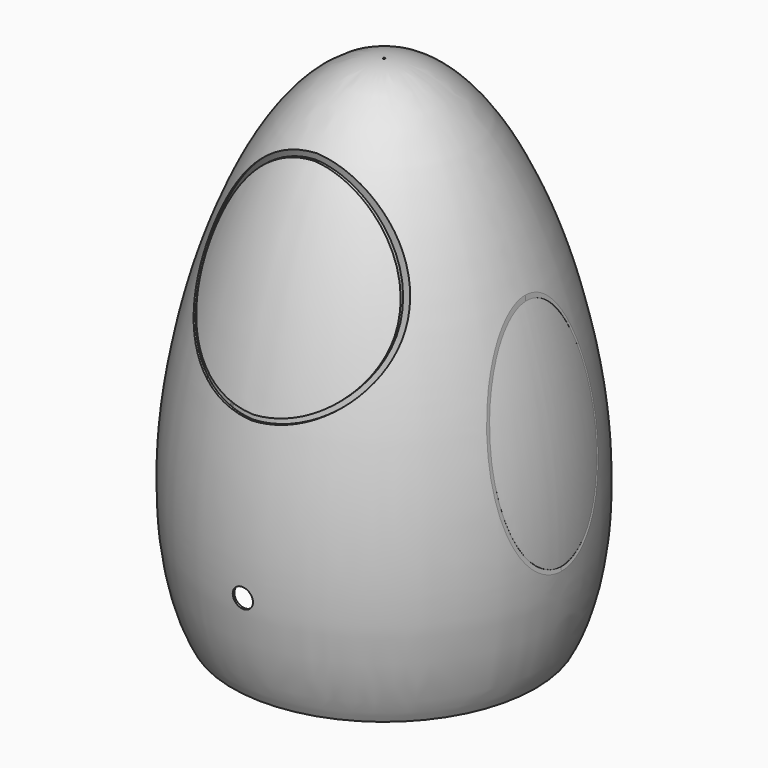
from build123d import *

# Parameters (mm, degrees)
F6_DEPTH       = 176.0365687371
F7_R           = 20
F8_DEPTH       = 15
F10_DEPTH      = 176.0365687371
F10_DEPTH_BACK = 176.0365687371
F12_DEPTH      = 176.0365687371
F12_DEPTH_BACK = 176.0365687371
F13_R          = 10
F14_DEPTH      = 100


# Not quite as in the source:
# - the dataset's text gives a spline's control points without its knots; the knots are read off the source's solid
# - the program builds the solid bodies; features that only make, move or delete a surface that nothing else refers to are left out


with BuildPart() as f4:
    # F2 (on Front) → F4 (revolve)
    with BuildSketch(Plane.XZ):
        with BuildLine():
            add(Edge.make_bspline(
                [(1, 449.0443005306), (80.1100924551, 451.0782588519), (193.5026632526, 197.5216639229), (177.718595848, 0), (150, -50.9556994694)],
                knots=[0, 0, 0, 0, 0.5180034602, 1, 1, 1, 1], degree=3))
            Line((1, 449.0443005306), (1.0514039698, 447.0449612318))
            add(Edge.make_bspline(
                [(1.0514039698, 447.0449612318), (5.6889924562, 447.1641958503), (14.8146657678, 446.4599738755), (28.0818566532, 442.7588814458), (40.9340638175, 436.5780096507), (57.4933039947, 425.253477856), (77.0343246982, 405.7570843458), (98.3770754656, 375.3396271098), (117.4020772089, 339.4781493047), (131.1745767843, 306.3735527905), (140.8608088078, 278.7467501585), (147.4397218669, 257.6520230515), (153.3131918368, 236.3794941135), (157.6036419872, 218.6684679305), (160.6640307325, 204.6072717881), (163.4728613383, 190.6522845028), (166.5161124872, 173.4285279629), (169.4361062201, 153.1618789749), (172.3750814452, 126.7445649885), (174.3001264236, 94.9854795873), (173.9432956348, 59.3073823577), (171.0522793788, 26.4763680651), (165.7627686174, -3.090947369), (158.216194357, -28.9750937643), (151.7820830163, -43.4942412252), (148.2431168154, -50)],
                knots=[0, 0, 0, 0, 0.03125, 0.0625, 0.09375, 0.125, 0.1875, 0.25, 0.3125, 0.375, 0.40625, 0.4375, 0.46875, 0.5, 0.515625, 0.53125, 0.5625, 0.59375, 0.625, 0.6875, 0.75, 0.8125, 0.875, 0.9375, 1, 1, 1, 1], degree=3))
            Line((148.2431168154, -50), (150, -50.9556994694))
        make_face()
    revolve(axis=Axis((0, 0, 140.6808644533), (0, 0, 1)))

    # F5 (on Front) → F6 (cut, through all)
    with BuildSketch(Plane.XZ):
        with BuildLine():
            add(Edge.make_bspline(
                [(0, 400), (59.0140521526, 398.2927203178), (143.2820959516, 269.3665802261), (55.2223846316, 202.2753804922), (0, 200)],
                knots=[0, 0, 0, 0, 0.5248109679, 1, 1, 1, 1], degree=3))
            add(Edge.make_bspline(
                [(0, 400), (-59.0140521526, 398.2927203178), (-143.2820959516, 269.3665802261), (-55.2223846316, 202.2753804922), (0, 200)],
                knots=[0, 0, 0, 0, 0.5248109679, 1, 1, 1, 1], degree=3))
        make_face()
        with BuildLine():
            add(Edge.make_bspline(
                [(-0.0001205983, 394.9977653066), (-6.5310531824, 394.7960276482), (-19.2521705838, 392.663716092), (-37.0198522817, 384.9642174164), (-53.1715953389, 373.423361096), (-67.2769986996, 358.8303413408), (-78.945849914, 342.0125314277), (-86.3298122589, 326.8622632752), (-90.6611195591, 314.5041209951), (-93.0823387791, 305.229555905), (-94.6395134009, 296.0625109198), (-95.189746261, 288.6086395993), (-95.1680818457, 282.8120957412), (-94.8339775011, 277.1489767391), (-93.8311621578, 270.3054768515), (-91.7383515242, 262.4779212136), (-87.8135974939, 252.5699057646), (-80.8706601583, 241.2076578757), (-69.5404081562, 229.3647628823), (-55.4800886394, 219.5291304996), (-33.5466161089, 209.4390648711), (-13.9709797098, 205.5996877414), (-8.74626e-05, 205.0043884577)],
                knots=[0.0004581342, 0.0004581342, 0.0004581342, 0.0004581342, 0.0625, 0.125, 0.1875, 0.25, 0.3125, 0.375, 0.40625, 0.4375, 0.46875, 0.5, 0.515625, 0.53125, 0.5625, 0.59375, 0.625, 0.6875, 0.75, 0.8125, 0.875, 0.9993890329, 0.9993890329, 0.9993890329, 0.9993890329], degree=3))
            add(Edge.make_bspline(
                [(-0.0001205793, 394.9977653056), (6.5308964276, 394.7960463513), (19.2520959342, 392.6637402976), (37.0198485436, 384.9642109116), (53.1715904201, 373.423355451), (67.2769929063, 358.8303366111), (78.9458434644, 342.0125276486), (86.3298053938, 326.8622603442), (90.6611124313, 314.5041188101), (93.0823314922, 305.2295543249), (94.6395059995, 296.0625100027), (95.1897388124, 288.6086392949), (95.1680743984, 282.8120959678), (94.8339700866, 277.1489775295), (93.8311548466, 270.3054783526), (91.7383444369, 262.4779235539), (87.8135908303, 252.5699091745), (80.8706542297, 241.2076624783), (69.5404033076, 229.3647685982), (55.4800849493, 219.529137014), (33.5465683901, 209.4390511181), (13.9708701194, 205.5996738585), (-8.74735e-05, 205.0043884574)],
                knots=[0.0004573712, 0.0004573712, 0.0004573712, 0.0004573712, 0.0625, 0.125, 0.1875, 0.25, 0.3125, 0.375, 0.40625, 0.4375, 0.46875, 0.5, 0.515625, 0.53125, 0.5625, 0.59375, 0.625, 0.6875, 0.75, 0.8125, 0.875, 0.9993895511, 0.9993895511, 0.9993895511, 0.9993895511], degree=3))
        make_face(mode=Mode.SUBTRACT)
    extrude(amount=F6_DEPTH, mode=Mode.SUBTRACT)

    # F9 (on Front) → F10 (cut, two sides)
    with BuildSketch(Plane.XZ) as f10_sk:
        with BuildLine():
            Line((137.2448259722, 324.7076010736), (136.2474411726, 324.6353268623))
            add(Edge.make_bspline(
                [(136.2474411726, 324.6353268623), (140.6513154507, 263.8618201017), (157.059520483, 150.0897556543), (182.0477843285, 26.0523948818)],
                knots=[0, 0, 0, 0, 302.0752202735, 302.0752202735, 302.0752202735, 302.0752202735], degree=3))
            Line((182.0477843285, 26.0523948818), (183.0280892625, 26.2498847203))
            add(Edge.make_bspline(
                [(137.2448259722, 324.7076010736), (138.3441848646, 309.5364379422), (142.0435898512, 272.5520944827), (155.0174901784, 177.4088911635), (170.5372786561, 88.2520786747), (183.0280892625, 26.2498847203)],
                knots=[0, 0, 0, 0, 0.25, 0.5, 1, 1, 1, 1], degree=3))
        make_face()
        with BuildLine():
            add(Edge.make_bspline(
                [(-136.2474411726, 324.6353268623), (-140.6513154507, 263.8618201017), (-157.059520483, 150.0897556543), (-182.0477843285, 26.0523948818)],
                knots=[0, 0, 0, 0, 302.0752202735, 302.0752202735, 302.0752202735, 302.0752202735], degree=3))
            Line((-136.2474411726, 324.6353268623), (-137.2448259722, 324.7076010736))
            add(Edge.make_bspline(
                [(-137.2448259722, 324.7076010736), (-138.3441848646, 309.5364379422), (-142.0435898512, 272.5520944827), (-155.0174901784, 177.4088911635), (-170.5372786561, 88.2520786747), (-183.0280892625, 26.2498847203)],
                knots=[0, 0, 0, 0, 0.25, 0.5, 1, 1, 1, 1], degree=3))
            Line((-183.0280892625, 26.2498847203), (-182.0477843285, 26.0523948818))
        make_face()
    extrude(amount=-F10_DEPTH, mode=Mode.SUBTRACT)
    extrude(f10_sk.sketch, amount=F10_DEPTH_BACK, mode=Mode.SUBTRACT)

    # F9 (on Front) → F12 (cut, two sides)
    with BuildSketch(Plane.XZ) as f12_sk:
        with BuildLine():
            Line((137.2448259722, 324.7076010736), (136.2474411726, 324.6353268623))
            add(Edge.make_bspline(
                [(136.2474411726, 324.6353268623), (140.6513154507, 263.8618201017), (157.059520483, 150.0897556543), (182.0477843285, 26.0523948818)],
                knots=[0, 0, 0, 0, 302.0752202735, 302.0752202735, 302.0752202735, 302.0752202735], degree=3))
            Line((182.0477843285, 26.0523948818), (183.0280892625, 26.2498847203))
            add(Edge.make_bspline(
                [(137.2448259722, 324.7076010736), (138.3441848646, 309.5364379422), (142.0435898512, 272.5520944827), (155.0174901784, 177.4088911635), (170.5372786561, 88.2520786747), (183.0280892625, 26.2498847203)],
                knots=[0, 0, 0, 0, 0.25, 0.5, 1, 1, 1, 1], degree=3))
        make_face()
        with BuildLine():
            add(Edge.make_bspline(
                [(-136.2474411726, 324.6353268623), (-140.6513154507, 263.8618201017), (-157.059520483, 150.0897556543), (-182.0477843285, 26.0523948818)],
                knots=[0, 0, 0, 0, 302.0752202735, 302.0752202735, 302.0752202735, 302.0752202735], degree=3))
            Line((-136.2474411726, 324.6353268623), (-137.2448259722, 324.7076010736))
            add(Edge.make_bspline(
                [(-137.2448259722, 324.7076010736), (-138.3441848646, 309.5364379422), (-142.0435898512, 272.5520944827), (-155.0174901784, 177.4088911635), (-170.5372786561, 88.2520786747), (-183.0280892625, 26.2498847203)],
                knots=[0, 0, 0, 0, 0.25, 0.5, 1, 1, 1, 1], degree=3))
            Line((-183.0280892625, 26.2498847203), (-182.0477843285, 26.0523948818))
        make_face()
    extrude(amount=-F12_DEPTH, mode=Mode.SUBTRACT)
    extrude(f12_sk.sketch, amount=F12_DEPTH_BACK, mode=Mode.SUBTRACT)

    # F13 (on offset) → F14 (cut)
    with BuildSketch(Plane.XZ.offset(200)):
        with Locations((0, 50)):
            Circle(F13_R)
    extrude(amount=-F14_DEPTH, mode=Mode.SUBTRACT)


with BuildPart() as f8:
    # F7 (on offset) → F8 (new body)
    with BuildSketch(Plane.XZ.offset(100)):
        with Locations((-40, 300)):
            Circle(F7_R)
    extrude(amount=F8_DEPTH)


with BuildPart() as f8b:
    # F7 (on offset) → F8, piece 2 (new body)
    with BuildSketch(Plane.XZ.offset(100)):
        with Locations((40, 300)):
            Circle(F7_R)
    extrude(amount=F8_DEPTH)


solid = Compound([f4.part, f8.part, f8b.part])
